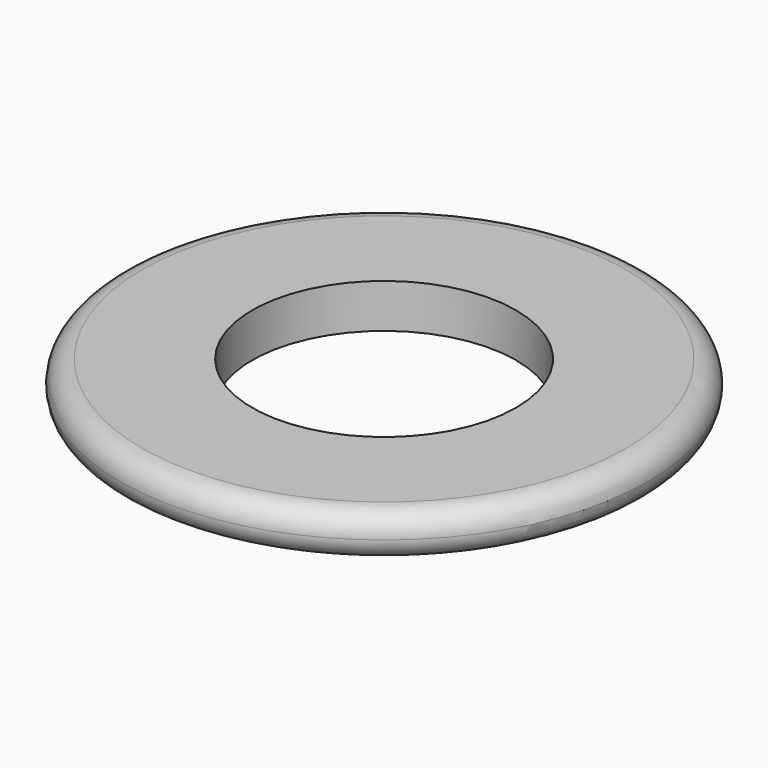
from build123d import *

# Parameters (mm, degrees)
F0_R     = 9
F0_R_2   = 4.5
F1_DEPTH = 1.5
F2_R     = 0.74999


# Not quite as in the source:
# - a fillet or chamfer is up to 0.001 mm smaller than in the source, because OpenCascade refuses the exact size


with BuildPart() as f1:
    # F0 (on Top) → F1 (new body)
    with BuildSketch(Plane.XY):
        Circle(F0_R)
        Circle(F0_R_2, mode=Mode.SUBTRACT)
    extrude(amount=F1_DEPTH)

    # F2 (radius 0.75 in the source; OpenCascade refuses exactly that, so slightly less here)
    f2_edges = [f1.edges().sort_by_distance(p)[0] for p in [
        (-9, 0, 1.5),
        (-9, 0, 0),
    ]]
    fillet(f2_edges, radius=F2_R)


solid = f1.part
